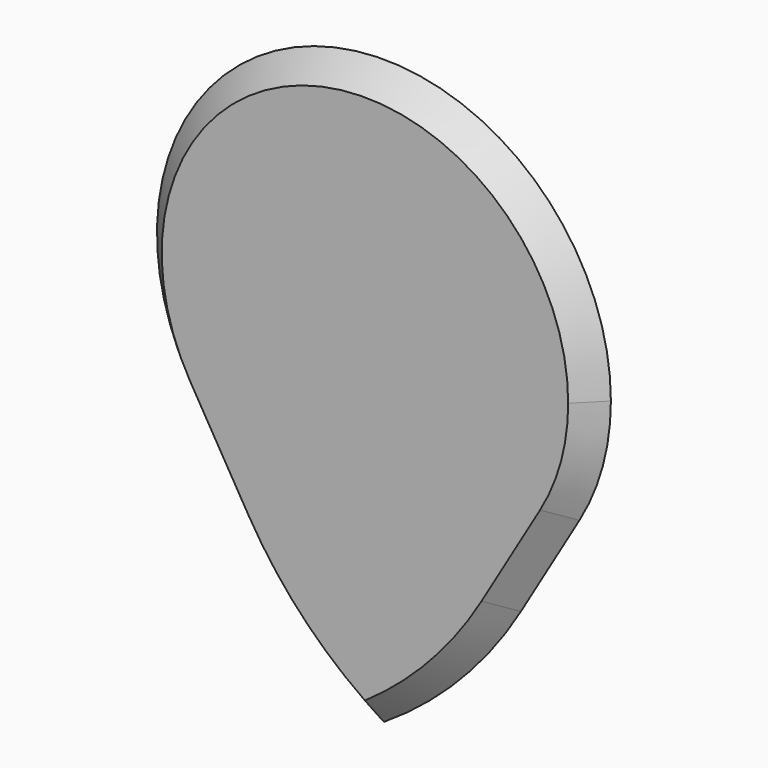
from build123d import *

# Parameters (mm, degrees)
F1_DEPTH               = 5
DRAFT_F1_DRAFTED_ANGLE = 45


# Not quite as in the source:
# - an extrude with a draft is written as a straight extrude whose walls are then drafted


with BuildPart() as f1:
    # F0 (on Front) → F1 (new body)
    with BuildSketch(Plane.XZ):
        with BuildLine():
            ThreePointArc((41.199747473, -24.2926478386), (46.1414577488, -12.5903855247), (47.828359065, 0))
            ThreePointArc((47.828359065, 0), (-12.5903855247, 46.1414577488), (-41.199747473, -24.2926478386))
            ThreePointArc((-41.199747473, -24.2926478386), (0, -47.828359065), (41.199747473, -24.2926478386))
        make_face()
        with BuildLine():
            ThreePointArc((41.199747473, -24.2926478386), (0, -47.828359065), (-41.199747473, -24.2926478386))
            Line((-41.199747473, -24.2926478386), (-28.8611945612, -45.2185373311))
            ThreePointArc((-28.8611945612, -45.2185373311), (-16.1970118349, -61.8607762226), (0, -75.089625268))
            ThreePointArc((0, -75.089625268), (16.1970118349, -61.8607762226), (28.8611945612, -45.2185373311))
            Line((28.8611945612, -45.2185373311), (41.199747473, -24.2926478386))
        make_face()
    extrude(amount=F1_DEPTH)

    # draft_F1_drafted
    draft_f1_drafted_walls = [f1.faces().sort_by_distance(p)[0] for p in [
        (0, -3.3333333333, 47.828359065),
        (-35.0304710171, -3.3333333333, -34.7555925848),
        (-16.1970118349, -3.3333333333, -61.8607762226),
        (16.1970118349, -3.3333333333, -61.8607762226),
        (35.0304710171, -3.3333333333, -34.7555925848),
    ]]
    draft(draft_f1_drafted_walls, neutral_plane=Plane.XZ, angle=DRAFT_F1_DRAFTED_ANGLE)


solid = f1.part
